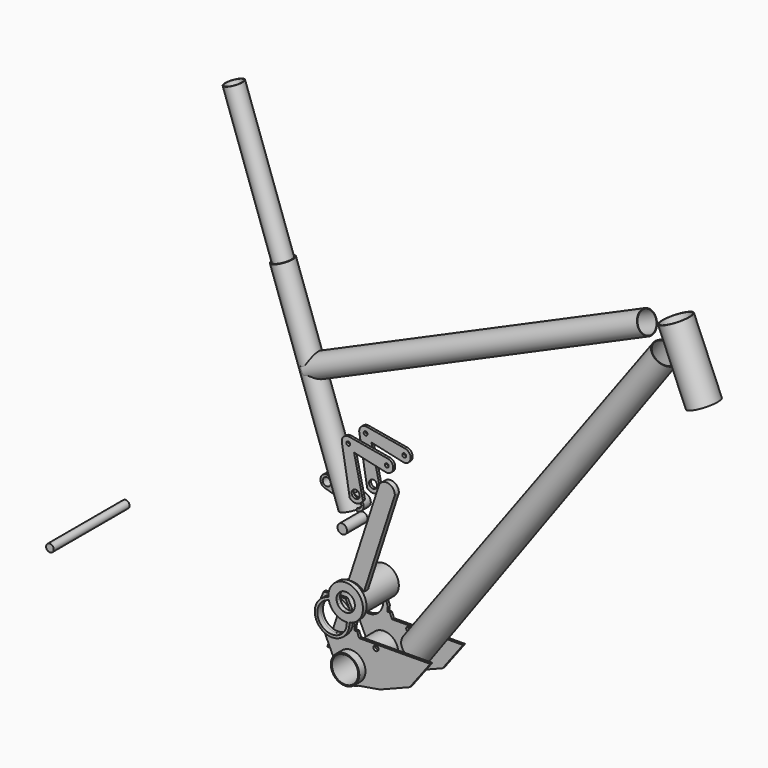
from build123d import *

# Parameters (mm, degrees)
F5_R      = 22.27
F5_R_2    = 20.5
F6_DEPTH  = 46
F7_R      = 23
F7_R_2    = 22
F8_DEPTH  = 34
F9_R      = 4
F9_R_2    = 22.27
F10_DEPTH = 4
F12_DEPTH = 7
F13_R     = 6
F14_DEPTH = 74
F21_R     = 7.5
F22_DEPTH = 20
F24_R     = 6.35
F24_R_2   = 3
F25_DEPTH = 4
F30_DEPTH = 8
F31_R     = 6.35
F32_DEPTH = 7


with BuildPart() as f2:
    # F1 (on Front) → F2 (revolve)
    with BuildSketch(Plane.XZ):
        Polygon((501.2564037907, 593.0426023652), (500.251106776, 592.5960848268), (543.8609052794, 489.8578378494), (544.8733216983, 490.2875831227), align=None)
    revolve(axis=Axis((501.8048992517, 0, 532.6308765113), (-0.3907311285, 0, 0.9205048535)))


with BuildPart() as f4:
    # F3 (on Front) → F4 (revolve)
    with BuildSketch(Plane.XZ):
        Polygon((92.7806691383, -12.3316956712), (93.5079050699, -12.8592034672), (479.5611913158, 519.3638715283), (478.8653748114, 519.9346949618), align=None)
    revolve(axis=Axis((262.6120625056, 0, 255.9247842068), (0.5898781878, 0, 0.8074922437)))


with BuildPart() as f6:
    # F5 (on Front) → F6 (new body, symmetric)
    with BuildSketch(Plane.XZ):
        with Locations((0, -36)):
            Circle(F5_R)
        with Locations((0, -36)):
            Circle(F5_R_2, mode=Mode.SUBTRACT)
    extrude(amount=F6_DEPTH, both=True)


with BuildPart() as f8:
    # F7 (on Front) → F8 (new body, symmetric)
    with BuildSketch(Plane.XZ):
        with Locations((-3, 53.8)):
            Circle(F7_R)
        with Locations((-3, 53.8)):
            Circle(F7_R_2, mode=Mode.SUBTRACT)
    extrude(amount=F8_DEPTH, both=True)


with BuildPart() as f10:
    # F9 (on face) → F10 (new body)
    with BuildSketch(Plane.XZ.offset(34)):
        with BuildLine():
            Line((-54.4824488461, 24.4921983182), (-25.9953716065, -36.4905660377))
            ThreePointArc((-25.9953716065, -36.4905660377), (-0.2452939356, -10.0011571241), (26, -36))
            ThreePointArc((26, -36), (22.1488363671, -49.6172334775), (11.7362271091, -59.2004520052))
            Line((11.7362271091, -59.2004520052), (44.8652207851, -53.6730534434))
            Line((44.8652207851, -53.6730534434), (91.5725156665, -35.2207881436))
            Line((91.5725156665, -35.2207881436), (123.4795674682, 7.0656553805))
            Line((123.4795674682, 7.0656553805), (12.457696721, 6.3794028908))
            Line((12.457696721, 6.3794028908), (9.1925212291, 14.4869210199))
            Line((9.1925212291, 14.4869210199), (5.2361269481, 14.4869210199))
            Line((5.2361269481, 14.4869210199), (5.2361269481, 21.5503554791))
            Line((5.2361269481, 21.5503554791), (6.3478340243, 21.5503554791))
            Line((6.3478340243, 21.5503554791), (2.3669704488, 31.4349462732))
            ThreePointArc((2.3669704488, 31.4349462732), (2.2008704423, 31.3957382036), (2.0344840784, 31.3577637018))
            ThreePointArc((2.0344840784, 31.3577637018), (2.5331052071, 28.3974097054), (2.7, 25.4))
            ThreePointArc((2.7, 25.4), (-42.7977908886, 5.7319616575), (-25.9542023882, 52.3492785517))
            ThreePointArc((-25.9542023882, 52.3492785517), (-25.977225013, 52.7767059547), (-25.9922892554, 53.2044877854))
            Line((-25.9922892554, 53.2044877854), (-43.1153662503, 52.4349116683))
            Line((-43.1153662503, 52.4349116683), (-54.4824488461, 24.4921983182))
        make_face()
        with Locations((38.7, 1.1)):
            Circle(F9_R, mode=Mode.SUBTRACT)
        with BuildLine():
            ThreePointArc((26, -36), (-0.2452939356, -10.0011571241), (-25.9953716065, -36.4905660377))
            ThreePointArc((-25.9953716065, -36.4905660377), (-13.4076668594, -58.2763208225), (11.7362271091, -59.2004520052))
            ThreePointArc((11.7362271091, -59.2004520052), (22.1488363671, -49.6172334775), (26, -36))
        make_face()
        with Locations((0, -36)):
            Circle(F9_R_2, mode=Mode.SUBTRACT)
        with BuildLine():
            ThreePointArc((-25.351281981, 48.3759614858), (-25.7396908644, 50.3494262231), (-25.9542023882, 52.3492785517))
            ThreePointArc((-25.9542023882, 52.3492785517), (-42.7977908886, 5.7319616575), (2.7, 25.4))
            ThreePointArc((2.7, 25.4), (2.5331052071, 28.3974097054), (2.0344840784, 31.3577637018))
            ThreePointArc((2.0344840784, 31.3577637018), (0.0545626162, 31.0037361126), (-1.948718019, 30.8240385142))
            ThreePointArc((-1.948718019, 30.8240385142), (-1.4627553592, 28.1313471434), (-1.3, 25.4))
            ThreePointArc((-1.3, 25.4), (-40.1874244992, 8.7690125735), (-25.351281981, 48.3759614858))
        make_face()
        with BuildLine():
            ThreePointArc((-24.9549013795, 52.3920563163), (-25.4547499889, 52.3752952248), (-25.9542023882, 52.3492785517))
            ThreePointArc((-25.9542023882, 52.3492785517), (-25.7396908644, 50.3494262231), (-25.351281981, 48.3759614858))
            ThreePointArc((-25.351281981, 48.3759614858), (-24.8392618831, 48.3936773184), (-24.3269742151, 48.3999841824))
            ThreePointArc((-24.3269742151, 48.3999841824), (-24.7327943147, 50.3815718124), (-24.9549013795, 52.3920563163))
        make_face()
        with BuildLine():
            ThreePointArc((-1.948718019, 30.8240385142), (0.0545626162, 31.0037361126), (2.0344840784, 31.3577637018))
            ThreePointArc((2.0344840784, 31.3577637018), (1.9196134127, 31.8445226736), (1.7957464499, 32.3290704442))
            ThreePointArc((1.7957464499, 32.3290704442), (-0.196508652, 31.9793575653), (-2.2124624047, 31.8141003246))
            ThreePointArc((-2.2124624047, 31.8141003246), (-2.0750764471, 31.3205382413), (-1.948718019, 30.8240385142))
        make_face()
    extrude(amount=-F10_DEPTH)


with BuildPart() as f10b:
    # F9 (on face) → F10, piece 2 (new body)
    with BuildSketch(Plane.XZ.offset(34)):
        with BuildLine():
            Line((-8.9017897844, 53.9725997448), (-24.9931087812, 53.249394751))
            ThreePointArc((-24.9931087812, 53.249394751), (-24.9781859253, 52.8205392137), (-24.9549013795, 52.3920563163))
            ThreePointArc((-24.9549013795, 52.3920563163), (-11.5022904619, 49.174327132), (-1.4084466916, 39.7170104117))
            Line((-1.4084466916, 39.7170104117), (-8.9017897844, 53.9725997448))
        make_face()
    extrude(amount=-F10_DEPTH)


with BuildPart() as f12:
    # F11 (on face) → F12 (new body)
    with BuildSketch(Plane.XZ.offset(34)):
        with BuildLine():
            ThreePointArc((2.6263632302, 27.3927275774), (17.9870413257, 36.813414222), (24, 53.8))
            ThreePointArc((24, 53.8), (-3.997043827, 80.7815845274), (-29.9263632302, 51.8072724226))
            ThreePointArc((-29.9263632302, 51.8072724226), (-27.9503563651, 52.1521008223), (-25.9542023882, 52.3492785517))
            ThreePointArc((-25.9542023882, 52.3492785517), (-25.4547499889, 52.3752952248), (-24.9549013795, 52.3920563163))
            ThreePointArc((-24.9549013795, 52.3920563163), (-20.9853852308, 52.1957707285), (-17.0876884022, 51.4188885507))
            ThreePointArc((-17.0876884022, 51.4188885507), (-4.1947401818, 68.0374594696), (11.2875, 53.8))
            ThreePointArc((11.2875, 53.8), (7.6698388627, 44.2980425756), (-1.3511274568, 39.6079643607))
            Line((-1.3511274568, 39.6079643607), (0.4730740469, 36.1375417236))
            Line((0.4730740469, 36.1375417236), (1.0001970656, 34.8286811612))
            ThreePointArc((1.0001970656, 34.8286811612), (1.4283455725, 33.5885428559), (1.7957464499, 32.3290704442))
            ThreePointArc((1.7957464499, 32.3290704442), (1.9196134127, 31.8445226736), (2.0344840784, 31.3577637018))
            ThreePointArc((2.0344840784, 31.3577637018), (2.4041165717, 29.3862461198), (2.6263632302, 27.3927275774))
        make_face()
        with BuildLine():
            ThreePointArc((-25.9542023882, 52.3492785517), (-27.9503563651, 52.1521008223), (-29.9263632302, 51.8072724226))
            ThreePointArc((-29.9263632302, 51.8072724226), (-29.7041165717, 49.8137538802), (-29.3344840784, 47.8422362982))
            ThreePointArc((-29.3344840784, 47.8422362982), (-27.3545626162, 48.1962638874), (-25.351281981, 48.3759614858))
            ThreePointArc((-25.351281981, 48.3759614858), (-25.7396908644, 50.3494262231), (-25.9542023882, 52.3492785517))
        make_face()
        with BuildLine():
            ThreePointArc((-29.3344840784, 47.8422362982), (-29.7041165717, 49.8137538802), (-29.9263632302, 51.8072724226))
            ThreePointArc((-29.9263632302, 51.8072724226), (-41.286585778, 4.4129586743), (2.7, 25.4))
            ThreePointArc((2.7, 25.4), (2.6815845274, 26.397043827), (2.6263632302, 27.3927275774))
            ThreePointArc((2.6263632302, 27.3927275774), (0.6503563651, 27.0478991777), (-1.3457976118, 26.8507214483))
            ThreePointArc((-1.3457976118, 26.8507214483), (-1.3114522541, 26.1257220786), (-1.3, 25.4))
            ThreePointArc((-1.3, 25.4), (-38.6737063104, 7.4445950505), (-29.3344840784, 47.8422362982))
        make_face()
        with BuildLine():
            ThreePointArc((-1.3457976118, 26.8507214483), (0.6503563651, 27.0478991777), (2.6263632302, 27.3927275774))
            ThreePointArc((2.6263632302, 27.3927275774), (2.4041165717, 29.3862461198), (2.0344840784, 31.3577637018))
            ThreePointArc((2.0344840784, 31.3577637018), (0.0545626162, 31.0037361126), (-1.948718019, 30.8240385142))
            ThreePointArc((-1.948718019, 30.8240385142), (-1.5603091356, 28.8505737769), (-1.3457976118, 26.8507214483))
        make_face()
        with BuildLine():
            ThreePointArc((-25.351281981, 48.3759614858), (-27.3545626162, 48.1962638874), (-29.3344840784, 47.8422362982))
            ThreePointArc((-29.3344840784, 47.8422362982), (-19.2, 32.2), (-1.3457976118, 26.8507214483))
            ThreePointArc((-1.3457976118, 26.8507214483), (-1.5603091356, 28.8505737769), (-1.948718019, 30.8240385142))
            ThreePointArc((-1.948718019, 30.8240385142), (-2.0750764471, 31.3205382413), (-2.2124624047, 31.8141003246))
            ThreePointArc((-2.2124624047, 31.8141003246), (-3.9372492874, 36.0938479238), (-6.4815937475, 39.9431907992))
            ThreePointArc((-6.4815937475, 39.9431907992), (-11.5725, 42.37), (-15.3276905834, 46.5777634261))
            ThreePointArc((-15.3276905834, 46.5777634261), (-19.7354761926, 47.9425181027), (-24.3269742151, 48.3999841824))
            ThreePointArc((-24.3269742151, 48.3999841824), (-24.8392618831, 48.3936773184), (-25.351281981, 48.3759614858))
        make_face()
        with BuildLine():
            ThreePointArc((-24.9549013795, 52.3920563163), (-25.4547499889, 52.3752952248), (-25.9542023882, 52.3492785517))
            ThreePointArc((-25.9542023882, 52.3492785517), (-25.7396908644, 50.3494262231), (-25.351281981, 48.3759614858))
            ThreePointArc((-25.351281981, 48.3759614858), (-24.8392618831, 48.3936773184), (-24.3269742151, 48.3999841824))
            ThreePointArc((-24.3269742151, 48.3999841824), (-24.7327943147, 50.3815718124), (-24.9549013795, 52.3920563163))
        make_face()
        with BuildLine():
            ThreePointArc((-1.948718019, 30.8240385142), (0.0545626162, 31.0037361126), (2.0344840784, 31.3577637018))
            ThreePointArc((2.0344840784, 31.3577637018), (1.9196134127, 31.8445226736), (1.7957464499, 32.3290704442))
            ThreePointArc((1.7957464499, 32.3290704442), (-0.196508652, 31.9793575653), (-2.2124624047, 31.8141003246))
            ThreePointArc((-2.2124624047, 31.8141003246), (-2.0750764471, 31.3205382413), (-1.948718019, 30.8240385142))
        make_face()
        with BuildLine():
            ThreePointArc((-17.0876884022, 51.4188885507), (-20.9853852308, 52.1957707285), (-24.9549013795, 52.3920563163))
            ThreePointArc((-24.9549013795, 52.3920563163), (-24.7327943147, 50.3815718124), (-24.3269742151, 48.3999841824))
            ThreePointArc((-24.3269742151, 48.3999841824), (-19.7354761926, 47.9425181027), (-15.3276905834, 46.5777634261))
            ThreePointArc((-15.3276905834, 46.5777634261), (-16.4276649071, 48.9183536185), (-17.0876884022, 51.4188885507))
        make_face()
        with BuildLine():
            ThreePointArc((-2.2124624047, 31.8141003246), (-0.196508652, 31.9793575653), (1.7957464499, 32.3290704442))
            ThreePointArc((1.7957464499, 32.3290704442), (1.4283455725, 33.5885428559), (1.0001970656, 34.8286811612))
            Line((1.0001970656, 34.8286811612), (0.4730740469, 36.1375417236))
            Line((0.4730740469, 36.1375417236), (-1.3511274568, 39.6079643607))
            ThreePointArc((-1.3511274568, 39.6079643607), (-3.9315637093, 39.5429019325), (-6.4815937475, 39.9431907992))
            ThreePointArc((-6.4815937475, 39.9431907992), (-3.9372492874, 36.0938479238), (-2.2124624047, 31.8141003246))
        make_face()
    extrude(amount=F12_DEPTH)


with BuildPart() as f14:
    # F13 (on Front) → F14 (new body, symmetric)
    with BuildSketch(Plane.XZ):
        with Locations((-438.5247997548, 0)):
            Circle(F13_R)
    extrude(amount=F14_DEPTH, both=True)


with BuildPart() as f16:
    # F15 (on Front) → F16 (revolve)
    with BuildSketch(Plane.XZ):
        Polygon((428.0766033653, 579.5205516757), (427.7137526275, 580.3441652636), (-97.5386940343, 348.9392435747), (-97.1758432965, 348.1156299868), align=None)
    revolve(axis=Axis((172.1429603092, 0, 448.6269957666), (0.9151262087, 0, 0.4031674864)))


with BuildPart() as f18:
    # F17 (on Front) → F18 (revolve)
    with BuildSketch(Plane.XZ):
        Polygon((-118.2801804317, 470.9146662515), (-119.1293984173, 470.6166246221), (-11.7247712434, 164.5857478987), (-10.8755532578, 164.8837895281), align=None)
    revolve(axis=Axis((-118.4722799712, 0, 421.6368347424), (-0.331157366, 0, 0.9435755396)))


with BuildPart() as f20:
    # F19 (on Front) → F20 (revolve)
    with BuildSketch(Plane.XZ):
        Polygon((-197.9597801261, 688.2550969276), (-121.3089038614, 469.851705173), (-120.4596858757, 470.1497468023), (-197.1105621405, 688.553138557), align=None)
    revolve(axis=Axis((-118.4722799712, 0, 421.6368347424), (-0.331157366, 0, 0.9435755396)))


with BuildPart() as f22:
    # F21 (on Front) → F22 (new body, symmetric)
    with BuildSketch(Plane.XZ):
        with Locations((-25.2, 138.7)):
            Circle(F21_R)
    extrude(amount=F22_DEPTH, both=True)


with BuildPart() as f25:
    # F24 (on offset) → F25 (new body)
    with BuildSketch(Plane.XZ.offset(15)):
        with BuildLine():
            Line((45.0792866924, 257.7899803277), (-15.5202416132, 268.3301646587))
            ThreePointArc((-15.5202416132, 268.3301646587), (-23.9489070515, 265.2886389483), (-26.5571872744, 256.7159990983))
            Line((-26.5571872744, 256.7159990983), (-14.2158837989, 184.3445748091))
            ThreePointArc((-14.2158837989, 184.3445748091), (-3.0278027841, 180.3528228637), (6.3226862973, 187.6791858309))
            Line((6.3226862973, 187.6791858309), (-7.5712497346, 249.1488009691))
            Line((-7.5712497346, 249.1488009691), (39.7688210528, 238.6630054739))
            ThreePointArc((39.7688210528, 238.6630054739), (53.2355145715, 245.2247693667), (45.0792866924, 257.7899803277))
        make_face()
        with Locations((-5, 192.5)):
            Circle(F24_R, mode=Mode.SUBTRACT)
        with Locations((-16.7, 258.4)):
            Circle(F24_R_2, mode=Mode.SUBTRACT)
        with Locations((43.6, 247.9)):
            Circle(F24_R_2, mode=Mode.SUBTRACT)
    extrude(amount=F25_DEPTH)


with BuildPart() as f26_1:
    # F26: instance of F10
    add(f10.part.mirror(Plane.XZ))


with BuildPart() as f27_1:
    # F27: instance of F25
    add(f25.part.mirror(Plane.XZ))


with BuildPart() as f30:
    # F29 (on offset) → F30 (new body)
    with BuildSketch(Plane.XZ.offset(20)):
        with BuildLine():
            ThreePointArc((-9.0322718431, 76.2020467014), (4.1626253754, 75.8666444602), (15.0391202321, 68.3886990939))
            Line((15.0391202321, 68.3886990939), (63.2673916522, 216.9705475902))
            ThreePointArc((63.2673916522, 216.9705475902), (53.2866882107, 230.1164467671), (38.5281287756, 222.726316203))
            Line((38.5281287756, 222.726316203), (-9.0322718431, 76.2020467014))
        make_face()
    extrude(amount=F30_DEPTH)


with BuildPart() as f30b:
    # F29 (on offset) → F30, piece 2 (new body)
    with BuildSketch(Plane.XZ.offset(20)):
        with BuildLine():
            Line((-42.0305820056, -25.4592771825), (-16.4258035795, -28.5485620821))
            Line((-16.4258035795, -28.5485620821), (3.0322718431, 31.3979532986))
            ThreePointArc((3.0322718431, 31.3979532986), (-10.1626253754, 31.7333555398), (-21.0391202321, 39.2113009061))
            Line((-21.0391202321, 39.2113009061), (-42.0305820056, -25.4592771825))
        make_face()
    extrude(amount=F30_DEPTH)


with BuildPart() as f32:
    # F31 (on Front) → F32 (new body, symmetric)
    with BuildSketch(Plane.XZ):
        with BuildLine():
            ThreePointArc((-49.7, 186.9), (-52.9695910302, 179.5039473299), (-60.6403190197, 176.9443081536))
            Line((-60.6403190197, 176.9443081536), (-17.3789502986, 163.5455582412))
            ThreePointArc((-17.3789502986, 163.5455582412), (-21.3183840651, 176.2054929109), (-9.2283292506, 181.6482549692))
            Line((-9.2283292506, 181.6482549692), (-56.1934790382, 196.265057968))
            ThreePointArc((-56.1934790382, 196.265057968), (-51.4821776115, 192.598016777), (-49.7, 186.9))
        make_face()
        with BuildLine():
            Line((-56.1934790382, 196.265057968), (-57.272677692, 196.6009332754))
            ThreePointArc((-57.272677692, 196.6009332754), (-69.5563950047, 188.5886318457), (-60.6403190197, 176.9443081536))
            ThreePointArc((-60.6403190197, 176.9443081536), (-52.9695910302, 179.5039473299), (-49.7, 186.9))
            ThreePointArc((-49.7, 186.9), (-51.4821776115, 192.598016777), (-56.1934790382, 196.265057968))
        make_face()
        with Locations((-59.7, 186.9)):
            Circle(F31_R, mode=Mode.SUBTRACT)
        with BuildLine():
            ThreePointArc((-9.2283292506, 181.6482549692), (-21.3183840651, 176.2054929109), (-17.3789502986, 163.5455582412))
            Line((-17.3789502986, 163.5455582412), (-12.7627541365, 162.1158471675))
            ThreePointArc((-12.7627541365, 162.1158471675), (-5.3307766583, 164.832691648), (-2.2, 172.1))
            ThreePointArc((-2.2, 172.1), (-4.1465315704, 178.0280389888), (-9.2283292506, 181.6482549692))
        make_face()
        with Locations((-12.2, 172.1)):
            Circle(F31_R, mode=Mode.SUBTRACT)
    extrude(amount=F32_DEPTH, both=True)


solid = Compound([f2.part, f4.part, f6.part, f8.part, f10.part, f10b.part, f12.part, f14.part, f16.part, f18.part, f20.part, f22.part, f25.part, f26_1.part, f27_1.part, f30.part, f30b.part, f32.part])
